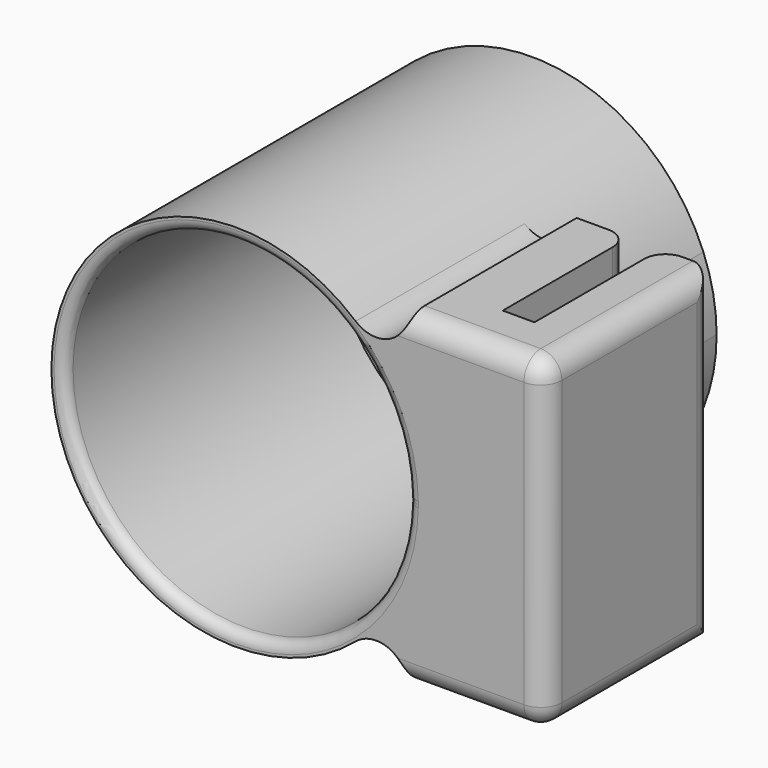
from build123d import *

# Parameters (mm, degrees)
F1_DEPTH    = 50.8
F0_W        = 12.7
F0_H        = 78.4147009254
F0_W_2      = 7.62
F2_DEPTH    = 12.7
F3_DEPTH    = 88.9
F5_DEPTH    = 88.9
F7_T1_DEPTH = 50.8
F8_R        = 5.08
F9_R        = 2.54
F11_R       = 44.45
F12_DEPTH   = 8.89


# Not quite as in the source:
# - a fillet or chamfer that OpenCascade refuses, or shapes differently, is made with other operations: its cross-section is extruded or revolved along the edge and cut away or added


with BuildPart() as f1:
    # F0 (on Front) → F1 (new body)
    with BuildSketch(Plane.XZ):
        with BuildLine():
            ThreePointArc((41.2700087631, 16.5102657972), (43.6477627692, 8.4068606055), (44.45, 0))
            ThreePointArc((44.45, 0), (43.6477627692, -8.4068606055), (41.2700087631, -16.5102657972))
            Line((41.2700087631, -16.5102657972), (41.2700087631, -39.2073504627))
            Line((41.2700087631, -39.2073504627), (53.9700087631, -39.2073504627))
            Line((53.9700087631, -39.2073504627), (53.9700087631, 39.2073504627))
            Line((53.9700087631, 39.2073504627), (41.2700087631, 39.2073504627))
            Line((41.2700087631, 39.2073504627), (41.2700087631, 16.5102657972))
        make_face()
    extrude(amount=-F1_DEPTH)



with BuildPart() as f1b:
    # F0 (on Front) → F1, piece 2 (new body)
    with BuildSketch(Plane.XZ):
        with Locations((67.9400087631, 0)):
            Rectangle(F0_W, F0_H)
    extrude(amount=-F1_DEPTH)


with BuildPart() as f1_1:
    add(f1.part)

    add(f1b.part)  # F2 merges F1b
    # F0 (on Front) → F2 (join)
    with BuildSketch(Plane.XZ):
        with Locations((57.7800087631, 0)):
            Rectangle(F0_W_2, F0_H)
    extrude(amount=-F2_DEPTH)

    # F0 (on Front) → F3 (join)
    with BuildSketch(Plane.XZ):
        with BuildLine():
            Line((41.2700087631, 0.6418735824), (41.2700087631, 16.5102657972))
            ThreePointArc((41.2700087631, 16.5102657972), (-44.45, 0), (41.2700087631, -16.5102657972))
            Line((41.2700087631, -16.5102657972), (41.2700087631, -0.6418735824))
            ThreePointArc((41.2700087631, -0.6418735824), (-41.275, 0), (41.2700087631, 0.6418735824))
        make_face()
    extrude(amount=-F3_DEPTH)

    # F4: union 

    # F0 (on Front) → F5 (join)
    with BuildSketch(Plane.XZ):
        with BuildLine():
            ThreePointArc((41.2700087631, -16.5102657972), (43.6477627692, -8.4068606055), (44.45, 0))
            ThreePointArc((44.45, 0), (43.6477627692, 8.4068606055), (41.2700087631, 16.5102657972))
            Line((41.2700087631, 16.5102657972), (41.2700087631, 0.6418735824))
            ThreePointArc((41.2700087631, 0.6418735824), (41.2737521719, 0.3209464941), (41.275, 0))
            ThreePointArc((41.275, 0), (41.2737521719, -0.3209464941), (41.2700087631, -0.6418735824))
            Line((41.2700087631, -0.6418735824), (41.2700087631, -16.5102657972))
        make_face()
    extrude(amount=-F5_DEPTH)

    # F6: union 

    # F7: fillet of radius 7.62 on 2 edges, made by hand

    # F7_s2 → F7_t1 (join)
    with BuildSketch(Plane.XZ.offset(-50.8)):
        with BuildLine():
            ThreePointArc((41.2700087631, -39.2073504627), (36.6353958241, -32.7032366386), (28.7404382359, -33.9085492171))
            ThreePointArc((28.7404382359, -33.9085492171), (36.0699423168, -25.9761768022), (41.2700087631, -16.5102657972))
            Line((41.2700087631, -16.5102657972), (41.2700087631, -39.2073504627))
        make_face()
        with BuildLine():
            ThreePointArc((28.7404382359, 33.9085492171), (36.6353958241, 32.7032366386), (41.2700087631, 39.2073504627))
            Line((41.2700087631, 39.2073504627), (41.2700087631, 16.5102657972))
            ThreePointArc((41.2700087631, 16.5102657972), (36.0699423168, 25.9761768022), (28.7404382359, 33.9085492171))
        make_face()
    extrude(amount=F7_T1_DEPTH)

    # F8
    f8_edges = [f1_1.edges().sort_by_distance(p)[0] for p in [
        (53.970009, 50.8, 0),
        (61.590009, 50.8, 0),
        (74.290009, 0, 0),
        (57.780009, 0, -39.20735),
        (57.780009, 0, 39.20735),
        (74.290009, 50.8, 0),
        (74.290009, 25.4, -39.20735),
        (74.290009, 25.4, 39.20735),
    ]]
    fillet(f8_edges, radius=F8_R)

    # F9
    f9_edges = [f1_1.edges().sort_by_distance(p)[0] for p in [
        (-41.270009, 0, -0.641874),
    ]]
    fillet(f9_edges, radius=F9_R)

    # F11 (on offset) → F12 (join)
    with BuildSketch(Plane(origin=(0, 88.9, 0), x_dir=(-1, 0, 0), z_dir=(0, 1, 0))):
        Circle(F11_R)
    extrude(amount=-F12_DEPTH)


solid = f1_1.part
